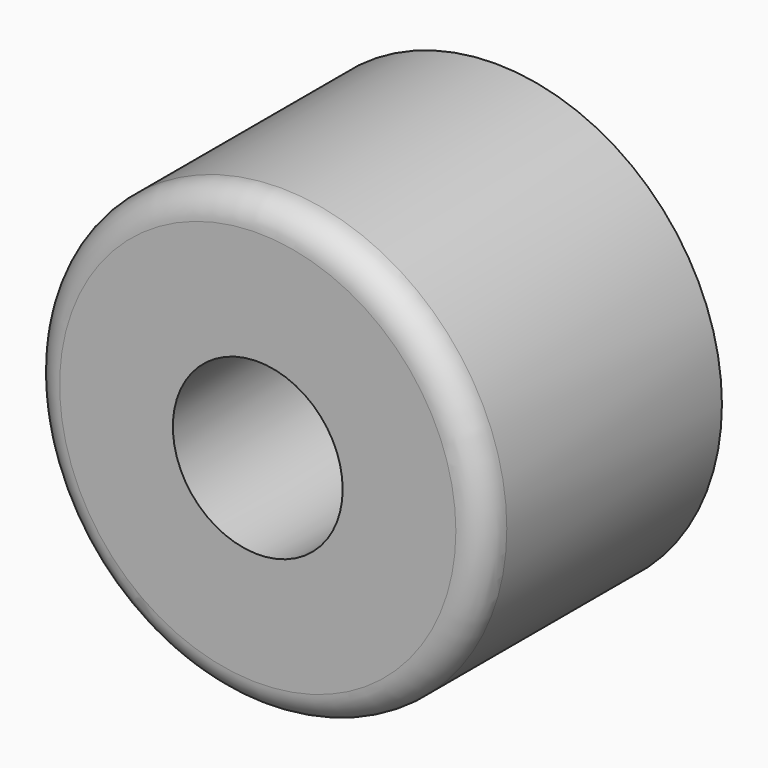
from build123d import *

# Parameters (mm, degrees)
F0_R           = 16
F1_DEPTH       = 21
F3_D           = 6
F3_DEPTH       = 21
F3_CBORE_D     = 12
F3_CBORE_DEPTH = 12
F3_TIP         = 1.8025818571
F4_R           = 2


with BuildPart() as f1:
    # F0 (on Front) → F1 (new body)
    with BuildSketch(Plane.XZ):
        Circle(F0_R)
    extrude(amount=F1_DEPTH)

    # F3
    with Locations(Plane.XZ.offset(21)):
        with Locations((0, 0)):
            CounterBoreHole(F3_D / 2, F3_CBORE_D / 2, F3_CBORE_DEPTH, depth=F3_DEPTH)
            with Locations((0, 0, -(F3_DEPTH + F3_TIP / 2))):  # 118° drill point
                Cone(0, F3_D / 2, F3_TIP, mode=Mode.SUBTRACT)

    # F4
    f4_edges = [f1.edges().sort_by_distance(p)[0] for p in [
        (-16, -21, 0),
    ]]
    fillet(f4_edges, radius=F4_R)


solid = f1.part
